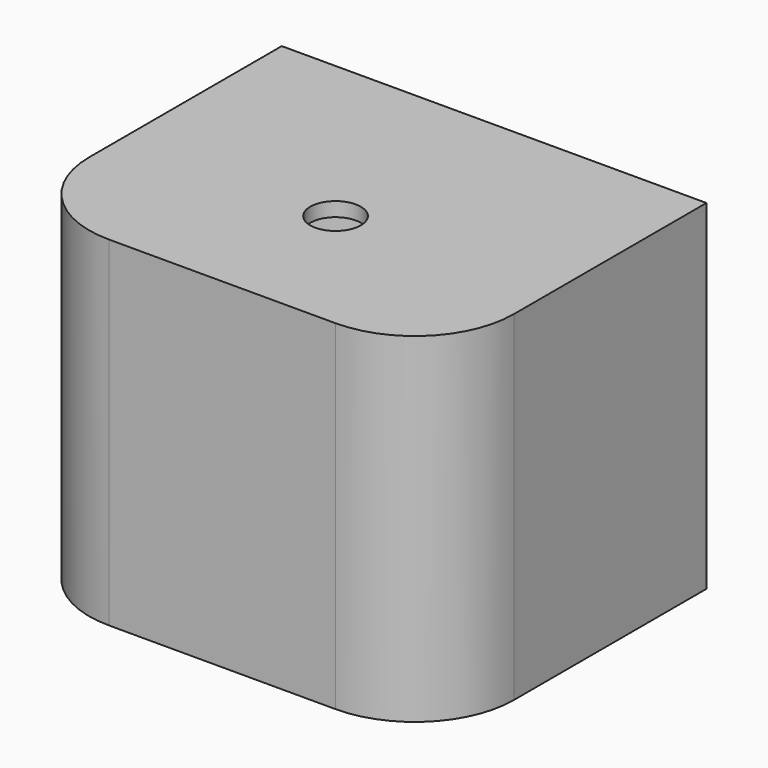
from build123d import *

# Parameters (mm, degrees)
F1_DEPTH = 24
F3_DEPTH = 23
F4_R     = 1.7859375
F5_DEPTH = 25
F7_DEPTH = 3
F8_R     = 1.25
F9_DEPTH = 5
F10_R    = 7


with BuildPart() as f1:
    # F0 (on Top) → F1 (new body)
    with BuildSketch(Plane.XY):
        Polygon((-15, -10), (15, -10), (15, 0), (15, 10), (15, 14), (-15, 14), (-15, 10), (-15, 0), align=None)
    extrude(amount=F1_DEPTH)

    # F2 (on Top) → F3 (cut)
    with BuildSketch(Plane.XY):
        with BuildLine():
            ThreePointArc((-8.2138157895, 0.7718355891), (-8.0544419216, 0.4004520472), (-8, 0))
            ThreePointArc((-8, 0), (-8.0544419216, -0.4004520472), (-8.2138157895, -0.7718355891))
            ThreePointArc((-8.2138157895, -0.7718355891), (0, -8.25), (8.2138157895, -0.7718355891))
            ThreePointArc((8.2138157895, -0.7718355891), (8, 0), (8.2138157895, 0.7718355891))
            ThreePointArc((8.2138157895, 0.7718355891), (0, 8.25), (-8.2138157895, 0.7718355891))
        make_face()
        with BuildLine():
            ThreePointArc((-8.2138157895, -0.7718355891), (-8.25, 0), (-8.2138157895, 0.7718355891))
            ThreePointArc((-8.2138157895, 0.7718355891), (-11, 0), (-8.2138157895, -0.7718355891))
        make_face()
        with BuildLine():
            ThreePointArc((-8.2138157895, -0.7718355891), (-8.0544419216, -0.4004520472), (-8, 0))
            ThreePointArc((-8, 0), (-8.0544419216, 0.4004520472), (-8.2138157895, 0.7718355891))
            ThreePointArc((-8.2138157895, 0.7718355891), (-8.25, 0), (-8.2138157895, -0.7718355891))
        make_face()
        with BuildLine():
            ThreePointArc((8.25, 0), (8.2409489825, 0.3863416473), (8.2138157895, 0.7718355891))
            ThreePointArc((8.2138157895, 0.7718355891), (8, 0), (8.2138157895, -0.7718355891))
            ThreePointArc((8.2138157895, -0.7718355891), (8.2409489825, -0.3863416473), (8.25, 0))
        make_face()
        with BuildLine():
            ThreePointArc((11, 0), (9.9004520472, 1.4455580784), (8.2138157895, 0.7718355891))
            ThreePointArc((8.2138157895, 0.7718355891), (8.2409489825, 0.3863416473), (8.25, 0))
            ThreePointArc((8.25, 0), (8.2409489825, -0.3863416473), (8.2138157895, -0.7718355891))
            ThreePointArc((8.2138157895, -0.7718355891), (9.9004520472, -1.4455580784), (11, 0))
        make_face()
    extrude(amount=F3_DEPTH, mode=Mode.SUBTRACT)

    # F4 (on face) → F5 (cut)
    with BuildSketch(Plane(origin=(0, 0, 23), x_dir=(1, 0, 0), z_dir=(0, 0, -1))):
        Circle(F4_R)
    extrude(amount=-F5_DEPTH, mode=Mode.SUBTRACT)

    # F6 (on face) → F7 (cut)
    with BuildSketch(Plane(origin=(0, 0, 0), x_dir=(1, 0, 0), z_dir=(0, 0, -1))):
        with BuildLine():
            ThreePointArc((8.8741196746, -9.5), (11.9240000791, -5.1786312974), (13, 0))
            ThreePointArc((13, 0), (11.9240000791, 5.1786312974), (8.8741196746, 9.5))
            Line((8.8741196746, 9.5), (8.8741196746, 1.3631851739))
            ThreePointArc((8.8741196746, 1.3631851739), (11, 0), (8.8741196746, -1.3631851739))
            Line((8.8741196746, -1.3631851739), (8.8741196746, -9.5))
        make_face()
        with BuildLine():
            Line((8.8741196746, 1.3631851739), (8.8741196746, 9.5))
            Line((8.8741196746, 9.5), (-8.8741196746, 9.5))
            Line((-8.8741196746, 9.5), (-8.8741196746, 1.3631851739))
            ThreePointArc((-8.8741196746, 1.3631851739), (-8.4992896122, 1.1173981921), (-8.2138157895, 0.7718355891))
            ThreePointArc((-8.2138157895, 0.7718355891), (0, 8.25), (8.2138157895, 0.7718355891))
            ThreePointArc((8.2138157895, 0.7718355891), (8.4992896122, 1.1173981921), (8.8741196746, 1.3631851739))
        make_face()
        with BuildLine():
            Line((-8.8741196746, -9.5), (8.8741196746, -9.5))
            Line((8.8741196746, -9.5), (8.8741196746, -1.3631851739))
            ThreePointArc((8.8741196746, -1.3631851739), (8.4992896122, -1.1173981921), (8.2138157895, -0.7718355891))
            ThreePointArc((8.2138157895, -0.7718355891), (0, -8.25), (-8.2138157895, -0.7718355891))
            ThreePointArc((-8.2138157895, -0.7718355891), (-8.4992896122, -1.1173981921), (-8.8741196746, -1.3631851739))
            Line((-8.8741196746, -1.3631851739), (-8.8741196746, -9.5))
        make_face()
        with BuildLine():
            Line((-8.8741196746, 1.3631851739), (-8.8741196746, 9.5))
            ThreePointArc((-8.8741196746, 9.5), (-13, 0), (-8.8741196746, -9.5))
            Line((-8.8741196746, -9.5), (-8.8741196746, -1.3631851739))
            ThreePointArc((-8.8741196746, -1.3631851739), (-11, 0), (-8.8741196746, 1.3631851739))
        make_face()
        with BuildLine():
            ThreePointArc((8.8741196746, -1.3631851739), (11, 0), (8.8741196746, 1.3631851739))
            Line((8.8741196746, 1.3631851739), (8.8741196746, -1.3631851739))
        make_face()
        with BuildLine():
            Line((8.8741196746, -1.3631851739), (8.8741196746, 1.3631851739))
            ThreePointArc((8.8741196746, 1.3631851739), (8.4992896122, 1.1173981921), (8.2138157895, 0.7718355891))
            ThreePointArc((8.2138157895, 0.7718355891), (0, 8.25), (-8.2138157895, 0.7718355891))
            ThreePointArc((-8.2138157895, 0.7718355891), (-8.4992896122, 1.1173981921), (-8.8741196746, 1.3631851739))
            Line((-8.8741196746, 1.3631851739), (-8.8741196746, -1.3631851739))
            ThreePointArc((-8.8741196746, -1.3631851739), (-8.4992896122, -1.1173981921), (-8.2138157895, -0.7718355891))
            ThreePointArc((-8.2138157895, -0.7718355891), (0, -8.25), (8.2138157895, -0.7718355891))
            ThreePointArc((8.2138157895, -0.7718355891), (8.4992896122, -1.1173981921), (8.8741196746, -1.3631851739))
        make_face()
        with BuildLine():
            Line((-8.8741196746, -1.3631851739), (-8.8741196746, 1.3631851739))
            ThreePointArc((-8.8741196746, 1.3631851739), (-11, 0), (-8.8741196746, -1.3631851739))
        make_face()
    extrude(amount=-F7_DEPTH, mode=Mode.SUBTRACT)

    # F8 (on face) → F9 (cut)
    with BuildSketch(Plane(origin=(0, 14, 0), x_dir=(-1, 0, 0), z_dir=(0, 1, 0))):
        with Locations((-10, 7)):
            Circle(F8_R)
        with Locations((10, 7)):
            Circle(F8_R)
    extrude(amount=-F9_DEPTH, mode=Mode.SUBTRACT)

    # F10
    f10_edges = [f1.edges().sort_by_distance(p)[0] for p in [
        (-15, -10, 12),
        (15, -10, 12),
    ]]
    fillet(f10_edges, radius=F10_R)


solid = f1.part
